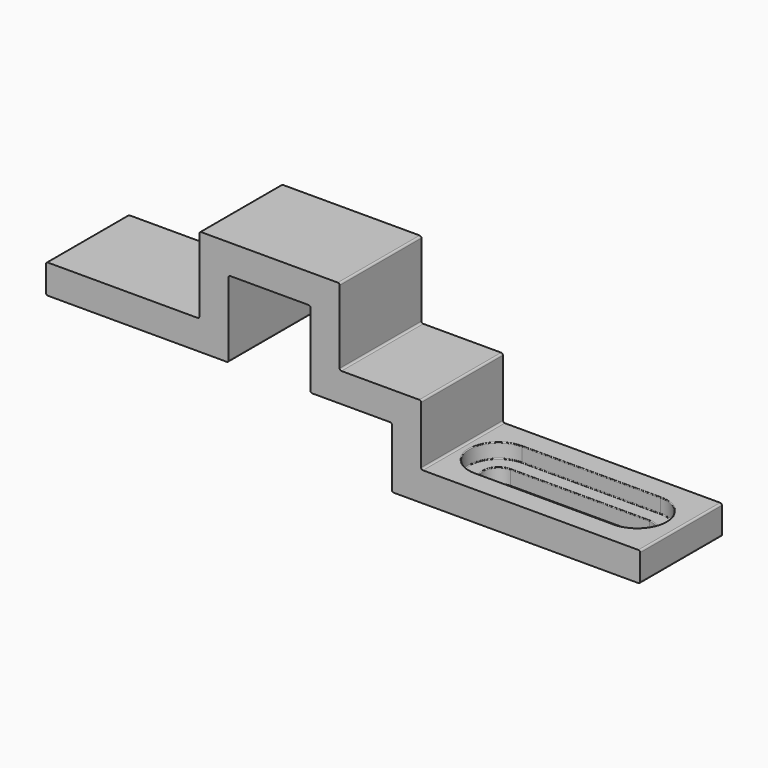
from build123d import *

# Parameters (mm, degrees)
F0_W      = 14
F0_H      = 4
F1_DEPTH  = 25
F2_W      = 4
F2_H      = 14
F3_DEPTH  = 10.50036
F4_W      = 14
F4_H      = 4
F5_DEPTH  = 15.21079
F6_W      = 4
F6_H      = 14
F7_DEPTH  = 10.50036
F8_W      = 14
F8_H      = 4
F9_DEPTH  = 11.159998
F10_W     = 4
F10_H     = 14
F11_DEPTH = 8.346948
F12_W     = 14
F12_H     = 4
F13_DEPTH = 30
F15_DEPTH = 3.9999999999
F17_DEPTH = 2
F18_R     = 0.1
F19_R     = 0.25


with BuildPart() as f1:
    # F0 (on Right) → F1 (new body)
    with BuildSketch(Plane.YZ):
        Rectangle(F0_W, F0_H)
    extrude(amount=F1_DEPTH)

    # F2 (on face) → F3 (join)
    with BuildSketch(Plane.XY.offset(2)):
        with Locations((23, 0)):
            Rectangle(F2_W, F2_H)
    extrude(amount=F3_DEPTH)

    # F4 (on face) → F5 (join)
    with BuildSketch(Plane.YZ.offset(25)):
        with Locations((0, 10.50036)):
            Rectangle(F4_W, F4_H)
    extrude(amount=F5_DEPTH)

    # F6 (on face) → F7 (join, through all)
    with BuildSketch(Plane(origin=(0, 0, 8.50036), x_dir=(1, 0, 0), z_dir=(0, 0, -1))):
        with Locations((38.21079, 0)):
            Rectangle(F6_W, F6_H)
    extrude(amount=F7_DEPTH)

    # F8 (on face) → F9 (join)
    with BuildSketch(Plane.YZ.offset(40.21079)):
        Rectangle(F8_W, F8_H)
    extrude(amount=F9_DEPTH)

    # F10 (on face) → F11 (join)
    with BuildSketch(Plane(origin=(0, 0, -2), x_dir=(1, 0, 0), z_dir=(0, 0, -1))):
        with Locations((49.370788, 0)):
            Rectangle(F10_W, F10_H)
    extrude(amount=F11_DEPTH)

    # F12 (on face) → F13 (join)
    with BuildSketch(Plane.YZ.offset(51.370788)):
        with Locations((0, -8.3469480001)):
            Rectangle(F12_W, F12_H)
    extrude(amount=F13_DEPTH)

    # F14 (on face) → F15 (cut, through all)
    with BuildSketch(Plane.XY.offset(-6.3469480001)):
        with BuildLine():
            ThreePointArc((56.370788, -2.0625), (57.8291957362, -1.4584077362), (58.433288, 0))
            ThreePointArc((58.433288, 0), (57.8291957362, 1.4584077362), (56.370788, 2.0625))
            ThreePointArc((56.370788, 2.0625), (54.308288, 0), (56.370788, -2.0625))
        make_face()
        with BuildLine():
            ThreePointArc((56.370788, 2.0625), (57.8291957362, 1.4584077362), (58.433288, 0))
            ThreePointArc((58.433288, 0), (57.8291957362, -1.4584077362), (56.370788, -2.0625))
            Line((56.370788, -2.0625), (75.370788, -2.0625))
            ThreePointArc((75.370788, -2.0625), (73.308288, 0), (75.370788, 2.0625))
            Line((75.370788, 2.0625), (56.370788, 2.0625))
        make_face()
        with BuildLine():
            ThreePointArc((77.433288, 0), (76.8291957362, 1.4584077362), (75.370788, 2.0625))
            ThreePointArc((75.370788, 2.0625), (73.308288, 0), (75.370788, -2.0625))
            ThreePointArc((75.370788, -2.0625), (76.8291957362, -1.4584077362), (77.433288, 0))
        make_face()
    extrude(amount=-F15_DEPTH, mode=Mode.SUBTRACT)

    # F16 (on face) → F17 (cut)
    with BuildSketch(Plane.XY.offset(-6.3469480001)):
        with BuildLine():
            ThreePointArc((56.370788, -4), (59.1992151247, -2.8284271247), (60.370788, 0))
            ThreePointArc((60.370788, 0), (59.1992151247, 2.8284271247), (56.370788, 4))
            ThreePointArc((56.370788, 4), (52.370788, 0), (56.370788, -4))
        make_face()
        with BuildLine():
            ThreePointArc((56.370788, 4), (59.1992151247, 2.8284271247), (60.370788, 0))
            ThreePointArc((60.370788, 0), (59.1992151247, -2.8284271247), (56.370788, -4))
            Line((56.370788, -4), (75.370788, -4))
            ThreePointArc((75.370788, -4), (71.370788, 0), (75.370788, 4))
            Line((75.370788, 4), (56.370788, 4))
        make_face()
        with BuildLine():
            ThreePointArc((79.370788, 0), (78.1992151247, 2.8284271247), (75.370788, 4))
            ThreePointArc((75.370788, 4), (71.370788, 0), (75.370788, -4))
            ThreePointArc((75.370788, -4), (78.1992151247, -2.8284271247), (79.370788, 0))
        make_face()
    extrude(amount=-F17_DEPTH, mode=Mode.SUBTRACT)

    # F18
    f18_edges = [f1.edges().sort_by_distance(p)[0] for p in [
        (52.370788, 0, -6.346948),
        (65.870788, 4, -6.346948),
        (79.370788, 0, -6.346948),
        (65.870788, -4, -6.346948),
        (65.870788, 4, -8.346948),
        (52.370788, 0, -8.346948),
        (54.308288, 0, -8.346948),
        (65.870788, 2.0625, -8.346948),
        (77.433288, 0, -8.346948),
        (79.370788, 0, -8.346948),
        (65.870788, -4, -8.346948),
        (65.870788, -2.0625, -8.346948),
    ]]
    fillet(f18_edges, radius=F18_R)

    # F19
    f19_edges = [f1.edges().sort_by_distance(p)[0] for p in [
        (51.370788, 0, -6.346948),
        (51.370788, 0, 2),
        (40.21079, 0, 2),
        (40.21079, 0, 12.50036),
        (21, 0, 2),
        (21, 0, 12.50036),
        (0, 0, 2),
        (0, 0, -2),
        (25, 0, -2),
        (25, 0, 8.50036),
        (36.21079, 0, 8.50036),
        (47.370788, 0, -2),
        (47.370788, 0, -10.346948),
        (81.370788, 0, -10.346948),
        (81.370788, 0, -6.346948),
        (36.21079, 0, -2),
    ]]
    fillet(f19_edges, radius=F19_R)


solid = f1.part
